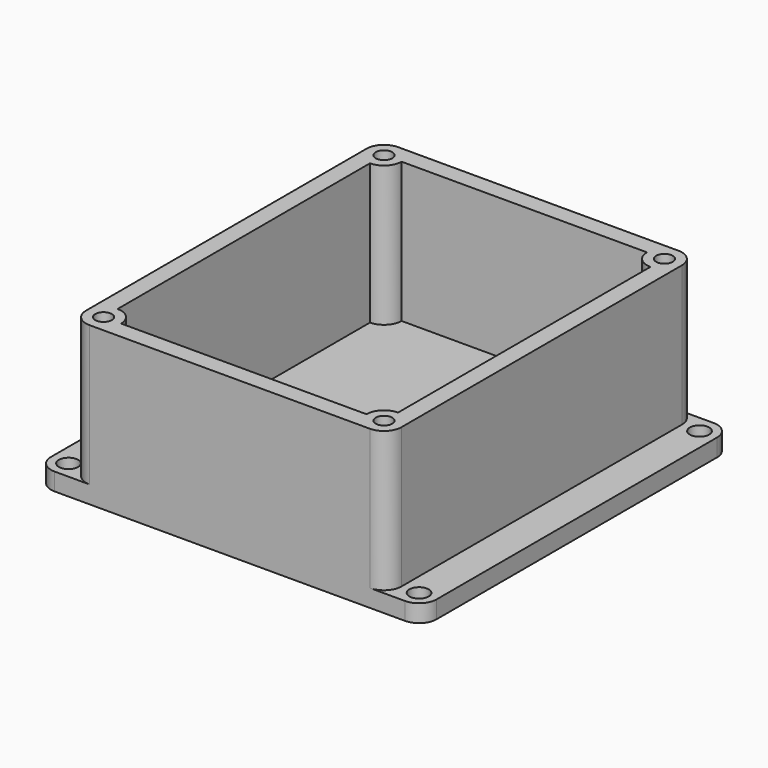
from build123d import *

# Parameters (mm, degrees)
F0_W          = 69.85
F0_H          = 69.85
F1_DEPTH      = 3.175
F2_R          = 3.175
F3_R          = 1.7499965
F4_DEPTH      = 25.4
F4_DEPTH_BACK = 101
F6_DEPTH      = 25.4
F7_R          = 1.499997
F8_DEPTH      = 6.35
F10_W         = 44.45
F10_H         = 57.15
F11_DEPTH     = 1.27
F12_W         = 8.9916
F12_H         = 14.4018
F13_DEPTH     = 10.9982


# Not quite as in the source:
# - an extrude ends at something that could not be found from the text; its depth is read off the source's solid


with BuildPart() as f1:
    # F0 (on Top) → F1 (new body)
    with BuildSketch(Plane.XY):
        Rectangle(F0_W, F0_H)
    extrude(amount=F1_DEPTH)

    # F2
    f2_edges = [f1.edges().sort_by_distance(p)[0] for p in [
        (-34.925, -34.925, 1.5875),
        (34.925, -34.925, 1.5875),
        (34.925, 34.925, 1.5875),
        (-34.925, 34.925, 1.5875),
    ]]
    fillet(f2_edges, radius=F2_R)

    # F3 (on face) → F4 (cut, two sides)
    with BuildSketch(Plane.XY.offset(3.175)) as f4_sk:
        with Locations((-31.75, 31.75)):
            Circle(F3_R)
        with Locations((31.75, 31.75)):
            Circle(F3_R)
        with Locations((31.75, -31.75)):
            Circle(F3_R)
        with Locations((-31.75, -31.75)):
            Circle(F3_R)
    extrude(amount=-F4_DEPTH, mode=Mode.SUBTRACT)
    extrude(f4_sk.sketch, amount=F4_DEPTH_BACK, mode=Mode.SUBTRACT)

    # F5 (on face) → F6 (join)
    with BuildSketch(Plane.XY.offset(3.175)):
        with BuildLine():
            Line((25.4, 34.925), (-25.4, 34.925))
            ThreePointArc((-25.4, 34.925), (-27.6450640303, 33.9950640303), (-28.575, 31.75))
            Line((-28.575, 31.75), (-28.575, -31.75))
            ThreePointArc((-28.575, -31.75), (-27.6450640303, -33.9950640303), (-25.4, -34.925))
            Line((-25.4, -34.925), (25.4, -34.925))
            ThreePointArc((25.4, -34.925), (27.6450640303, -33.9950640303), (28.575, -31.75))
            Line((28.575, -31.75), (28.575, 31.75))
            ThreePointArc((28.575, 31.75), (27.6450640303, 33.9950640303), (25.4, 34.925))
        make_face()
        with BuildLine():
            ThreePointArc((-25.4, 28.575), (-23.1549359697, 29.5049359697), (-22.225, 31.75))
            Line((-22.225, 31.75), (22.225, 31.75))
            ThreePointArc((22.225, 31.75), (23.1549359697, 29.5049359697), (25.4, 28.575))
            Line((25.4, 28.575), (25.4, -28.575))
            ThreePointArc((25.4, -28.575), (23.1549359697, -29.5049359697), (22.225, -31.75))
            Line((22.225, -31.75), (-22.225, -31.75))
            ThreePointArc((-22.225, -31.75), (-23.1549359697, -29.5049359697), (-25.4, -28.575))
            Line((-25.4, -28.575), (-25.4, 28.575))
        make_face(mode=Mode.SUBTRACT)
    extrude(amount=F6_DEPTH)

    # F7 (on face) → F8 (cut)
    with BuildSketch(Plane.XY.offset(28.575)):
        with Locations((-25.4, 31.75)):
            Circle(F7_R)
        with Locations((25.4, 31.75)):
            Circle(F7_R)
        with Locations((25.4, -31.75)):
            Circle(F7_R)
        with Locations((-25.4, -31.75)):
            Circle(F7_R)
    extrude(amount=-F8_DEPTH, mode=Mode.SUBTRACT)


with BuildPart() as f11:
    # F10 (on offset) → F11 (new body)
    with BuildSketch(Plane.XY.offset(6.35)):
        with Locations((0.3046067432, 0.0383506862)):
            Rectangle(F10_W, F10_H)
    extrude(amount=F11_DEPTH)

    # F12 (on face) → F13 (join)
    with BuildSketch(Plane.XY.offset(7.62)):
        with Locations((-12.7947921936, -21.3357493138)):
            Rectangle(F12_W, F12_H)
    extrude(amount=F13_DEPTH)


solid = f1.part
